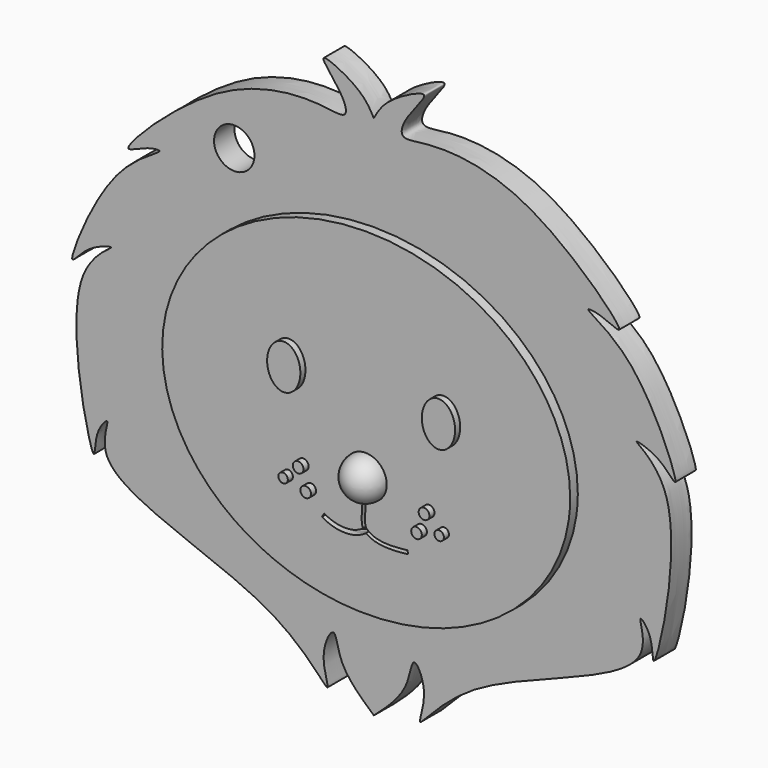
from build123d import *

# Parameters (mm, degrees)
F1_DEPTH  = 4
F3_DEPTH  = 1.5
F7_DEPTH  = 1
F8_R      = 0.8434589126
F8_R_2    = 0.7451557878
F8_R_3    = 0.8331091663
F9_DEPTH  = 1
F11_D     = 6.35
F13_DEPTH = 1
F14_DEPTH = 1


# Not quite as in the source:
# - ends of sketch curves that miss each other by under 0.0002 mm in the source are joined
# - the dataset's text gives a spline's control points without its knots; the knots are read off the source's solid


with BuildPart() as f1:
    # F0 (on Front) → F1 (new body)
    with BuildSketch(Plane.XZ):
        with BuildLine():
            add(Edge.make_bspline(
                [(0, 48.9745251834), (0.5905240779, 50.0606643379), (1.860875099, 52.3971956253), (10.1604689545, 56.4065843429), (5.0538324692, 51.1953719423), (3.6841452297, 47.2350083151), (9.3357678376, 48.605493595), (24.3329752849, 47.7431180711), (41.8781156231, 30.0061723136), (35.924093302, 33.4134701449), (31.8351204996, 33.8501917737), (41.9047611955, 29.8284598447), (49.2866484075, 10.6233912762), (45.2987628842, 16.7224406114), (38.6966212633, 18.5775084886), (50.4464264996, 13.3142921545), (43.4609717324, -16.9896703334), (44.0233204496, -8.5527794206), (40.8329577777, -5.0865522771), (45.8026866177, -15.5333206311), (14.8522287096, -21.5937486656), (5.7839163713, -35.1680373412), (8.7772886061, -27.9317621535), (5.992076876, -22.4937004561), (5.618991097, -28.6774050245), (2.1058790474, -31.8160447921), (0, -33.6974523962)],
                knots=[0, 0, 0, 0, 0.0328673193, 0.0707050469, 0.1038560693, 0.1320618367, 0.1623011415, 0.2272260769, 0.2953814591, 0.3222684226, 0.3454810209, 0.3908555213, 0.4542698663, 0.482730907, 0.5142049633, 0.5571542136, 0.6343634166, 0.6622400057, 0.6878428911, 0.7227602299, 0.8091537485, 0.8611415344, 0.8939691042, 0.9254431764, 0.9553080999, 1, 1, 1, 1], degree=3))
            add(Edge.make_bspline(
                [(0, 48.9745251834), (-0.5905240779, 50.0606643379), (-1.860875099, 52.3971956253), (-10.1604689545, 56.4065843429), (-5.0538324692, 51.1953719423), (-3.6841452297, 47.2350083151), (-9.3357678376, 48.605493595), (-24.3329752849, 47.7431180711), (-41.8781156231, 30.0061723136), (-35.924093302, 33.4134701449), (-31.8351204996, 33.8501917737), (-41.9047611955, 29.8284598447), (-49.2866484075, 10.6233912762), (-45.2987628842, 16.7224406114), (-38.6966212633, 18.5775084886), (-50.4464264996, 13.3142921545), (-43.4609717324, -16.9896703334), (-44.0233204496, -8.5527794206), (-40.8329577777, -5.0865522771), (-45.8026866177, -15.5333206311), (-14.8522287096, -21.5937486656), (-5.7839163713, -35.1680373412), (-8.7772886061, -27.9317621535), (-5.992076876, -22.4937004561), (-5.618991097, -28.6774050245), (-2.1058790474, -31.8160447921), (0, -33.6974523962)],
                knots=[0, 0, 0, 0, 0.0328673193, 0.0707050469, 0.1038560693, 0.1320618367, 0.1623011415, 0.2272260769, 0.2953814591, 0.3222684226, 0.3454810209, 0.3908555213, 0.4542698663, 0.482730907, 0.5142049633, 0.5571542136, 0.6343634166, 0.6622400057, 0.6878428911, 0.7227602299, 0.8091537485, 0.8611415344, 0.8939691042, 0.9254431764, 0.9553080999, 1, 1, 1, 1], degree=3))
        make_face()
    extrude(amount=F1_DEPTH)

    # F2 (on face) → F3 (join)
    with BuildSketch(Plane.XZ.offset(4)):
        with BuildLine():
            add(Edge.make_bspline(
                [(32.073777169, 7.431156002), (32.073777169, 53.2980368481), (-16.0368885845, 30.3645964251), (-64.147554338, 7.431156002), (-16.0368885845, -15.5022844211), (32.073777169, -38.4357248442), (32.073777169, 7.431156002)],
                knots=[0, 0, 0, 2.0943951024, 2.0943951024, 4.1887902048, 4.1887902048, 6.2831853072, 6.2831853072, 6.2831853072], degree=2, weights=[1, 0.5, 1, 0.5, 1, 0.5, 1]))
        make_face()
    extrude(amount=F3_DEPTH)

    # F6 (on face) → F7 (join)
    with BuildSketch(Plane.XZ.offset(5.5)):
        with BuildLine():
            add(Edge.make_bspline(
                [(-12.1630271897, 15.1178985834), (-16.6856053012, 15.1178985834), (-14.4243162454, 9.8631368019), (-12.1630271897, 4.6083750203), (-9.9017381339, 9.8631368019), (-7.6404490782, 15.1178985834), (-12.1630271897, 15.1178985834)],
                knots=[0, 0, 0, 2.0943951024, 2.0943951024, 4.1887902048, 4.1887902048, 6.2831853072, 6.2831853072, 6.2831853072], degree=2, weights=[1, 0.5, 1, 0.5, 1, 0.5, 1]))
        make_face()
        with BuildLine():
            add(Edge.make_bspline(
                [(12.1630271897, 15.1178985834), (7.6404490782, 15.1178985834), (9.9017381339, 9.8631368019), (12.1630271897, 4.6083750203), (14.4243162454, 9.8631368019), (16.6856053012, 15.1178985834), (12.1630271897, 15.1178985834)],
                knots=[0, 0, 0, 2.0943951024, 2.0943951024, 4.1887902048, 4.1887902048, 6.2831853072, 6.2831853072, 6.2831853072], degree=2, weights=[1, 0.5, 1, 0.5, 1, 0.5, 1]))
        make_face()
    extrude(amount=F7_DEPTH)

    # F8 (on face) → F9 (join)
    with BuildSketch(Plane.XZ.offset(5.5)):
        with Locations((9.8962336779, -1.557180658)):
            Circle(F8_R)
        with Locations((12.2673036531, -3.7965250667)):
            Circle(F8_R_2)
        with Locations((8.7106991559, -4.5868819579)):
            Circle(F8_R_3)
        with Locations((-9.8962336779, -1.557180658)):
            Circle(F8_R)
        with Locations((-12.2673036531, -3.7965250667)):
            Circle(F8_R_2)
        with Locations((-8.7106991559, -4.5868819579)):
            Circle(F8_R_3)
    extrude(amount=F9_DEPTH)

    # F11 (through all)
    with Locations(Plane.XZ.offset(4)):
        with Locations((-21.9434686005, 37.6923754811)):
            Hole(F11_D / 2)

    # F12 (on face) → F13 (cut)
    with BuildSketch(Plane.XZ.offset(5.5)):
        with BuildLine():
            Line((0.5233820891, -0.102892056), (0, 0))
            add(Edge.make_bspline(
                [(0, 0), (-0.4881215915, -2.482933166), (-0.9613370757, -6.0718488601), (-0.5612955072, -7.208765739), (-0.5044280314, -7.318585159)],
                knots=[0, 0, 0, 0, 0.420157188, 0.4745929198, 0.4745929198, 0.4745929198, 0.4745929198], degree=3))
            add(Edge.make_bspline(
                [(-0.5044280314, -7.318585159), (-0.3839649909, -7.5512169235), (-0.2142195664, -7.6914798202), (0, -7.8503383877)],
                knots=[0.4745929198, 0.4745929198, 0.4745929198, 0.4745929198, 0.5899047683, 0.5899047683, 0.5899047683, 0.5899047683], degree=3))
            add(Edge.make_bspline(
                [(0, -7.8503383877), (0.7618507889, -8.4153032363), (2.0862101548, -9.2154659724), (6.5707527101, -8.6289253086)],
                knots=[0.5899047683, 0.5899047683, 0.5899047683, 0.5899047683, 1, 1, 1, 1], degree=3))
            Line((6.5707527101, -8.6289253086), (6.5015776088, -8.1000298636))
            add(Edge.make_bspline(
                [(0.5233820891, -0.102892056), (0.3797897829, -0.8333045303), (0.1731601234, -2.0220344332), (-0.0353459818, -3.5800416091), (-0.1460573612, -4.6810377313), (-0.199319377, -5.6585454397), (-0.1867127098, -6.3187377859), (-0.141191681, -6.7149895118), (-0.0939902885, -6.9252852479), (-0.0410382703, -7.060637948), (0.0131017546, -7.1503449609), (0.0805598098, -7.2295486825), (0.1662733588, -7.3058848998), (0.2568355886, -7.3766068571), (0.3644102935, -7.4568564767), (0.5056396611, -7.5580867604), (0.6919212974, -7.6773815015), (0.977065634, -7.8338758033), (1.4264666337, -8.0207895201), (2.1895483998, -8.2051613796), (3.5908418883, -8.3467889078), (5.15759163, -8.2758119904), (6.5015776088, -8.1000298636)],
                knots=[0, 0, 0, 0, 0.125, 0.1875, 0.25, 0.3125, 0.375, 0.40625, 0.4375, 0.46875, 0.5, 0.53125, 0.5625, 0.578125, 0.59375, 0.625, 0.65625, 0.6875, 0.75, 0.8125, 0.875, 1, 1, 1, 1], degree=3))
        make_face()
        with BuildLine():
            add(Edge.make_bspline(
                [(-0.5044280314, -7.318585159), (-0.3839649909, -7.5512169235), (-0.2142195664, -7.6914798202), (0, -7.8503383877)],
                knots=[0.4745929198, 0.4745929198, 0.4745929198, 0.4745929198, 0.5899047683, 0.5899047683, 0.5899047683, 0.5899047683], degree=3))
            Line((-0.5044280314, -7.318585159), (-0.5896776551, -7.4213962061))
            add(Edge.make_bspline(
                [(-0.5896776551, -7.4213962061), (-0.764080003, -7.5340299903), (-1.1746516134, -7.7652622598), (-1.8209211502, -8.0143530956), (-2.54743991, -8.1657381012), (-3.3162912457, -8.2123557487), (-4.1118400446, -8.1635665698), (-5.1915722143, -7.9505272579), (-6.027023617, -7.6025591287), (-6.593961875, -7.2623091615)],
                knots=[0.0337133983, 0.0337133983, 0.0337133983, 0.0337133983, 0.125, 0.25, 0.375, 0.5, 0.625, 0.75, 1, 1, 1, 1], degree=3))
            Line((-6.593961875, -7.2623091615), (-6.9468696602, -7.8503383877))
            add(Edge.make_bspline(
                [(0, -7.8503383877), (-1.0352784213, -8.5823494277), (-3.2074066813, -9.1627686895), (-5.6623036495, -8.6212751465), (-6.9468696602, -7.8503383877)],
                knots=[0, 0, 0, 0, 0.4813648874, 1, 1, 1, 1], degree=3))
        make_face()
    extrude(amount=-F13_DEPTH, mode=Mode.SUBTRACT)

    # F14 (cut): a face of the model
    f14_faces = [f1.faces().sort_by_distance(p)[0] for p in [
        (-0.479223587, -4.5, -6.8214875179),
    ]]
    extrude(f14_faces, amount=-F14_DEPTH, mode=Mode.SUBTRACT)


with BuildPart() as f5:
    # F4 (on Top) → F5 (revolve)
    with BuildSketch(Plane.XY):
        with BuildLine():
            Line((0, -5.6336116977), (0, -8.9680617675))
            ThreePointArc((0, -8.9680617675), (2.3578122559, -7.9914239536), (3.3344500698, -5.6336116977))
            Line((3.3344500698, -5.6336116977), (0, -5.6336116977))
        make_face()
    revolve(axis=Axis((0, -7.3008367326, 0), (0, 1, 0)))


solid = Compound([f1.part, f5.part])
